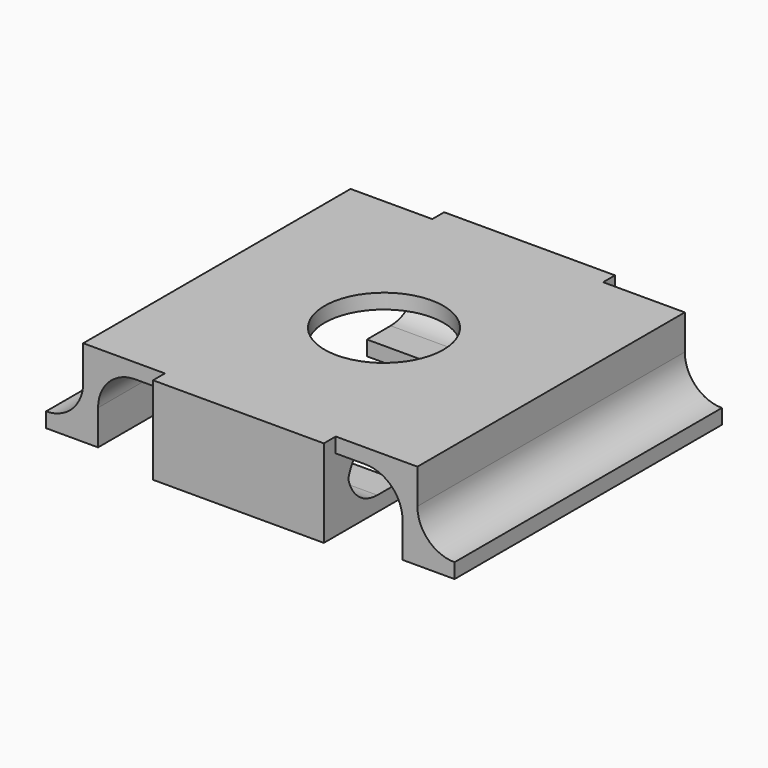
from build123d import *

# Parameters (mm, degrees)
F0_W         = 45
F0_H         = 45
F1_DEPTH     = 2
F2_R         = 8
F3_DEPTH     = 25
F4_W         = 23
F4_H         = 3.9995294809
F4_H_2       = 4
F5_DEPTH     = 9.8
F6_W         = 23
F6_H         = 9
F6_H_2       = 4
F7_DEPTH     = 2
F8_W         = 23
F8_H         = 13
F9_DEPTH     = 2
F10_W        = 2
F10_H        = 45
F11_DEPTH    = 7.7
F12_W        = 7
F12_H        = 45
F13_W        = 7
F13_H        = 45
F14_DEPTH    = 2
F15_T1_DEPTH = 23
F15_T3_DEPTH = 45


# Not quite as in the source:
# - a fillet or chamfer that OpenCascade refuses, or shapes differently, is made with other operations: its cross-section is extruded or revolved along the edge and cut away or added


with BuildPart() as f1:
    # F0 (on Top) → F1 (new body)
    with BuildSketch(Plane.XY):
        Rectangle(F0_W, F0_H)
    extrude(amount=F1_DEPTH)

    # F2 (on face) → F3 (cut)
    with BuildSketch(Plane.XY.offset(2)):
        Circle(F2_R)
    extrude(amount=-F3_DEPTH, mode=Mode.SUBTRACT)

    # F4 (on face) → F5 (join)
    with BuildSketch(Plane.XY.offset(2)):
        with Locations((0, 22.5)):
            Rectangle(F4_W, F4_H)
        with Locations((0, -22.5)):
            Rectangle(F4_W, F4_H_2)
    extrude(amount=-F5_DEPTH)

    # F6 (on face) → F7 (join)
    with BuildSketch(Plane(origin=(0, 0, -7.8), x_dir=(1, 0, 0), z_dir=(0, 0, -1))):
        with Locations((0, 16)):
            Rectangle(F6_W, F6_H)
        with Locations((0, 22.5)):
            Rectangle(F6_W, F6_H_2)
    extrude(amount=F7_DEPTH)

    # F8 (on face) → F9 (join)
    with BuildSketch(Plane(origin=(0, 0, -7.8), x_dir=(1, 0, 0), z_dir=(0, 0, -1))):
        with Locations((0, -17.9997647405)):
            Rectangle(F8_W, F8_H)
    extrude(amount=F9_DEPTH)

    # F10 (on face) → F11 (join)
    with BuildSketch(Plane(origin=(0, 0, 0), x_dir=(1, 0, 0), z_dir=(0, 0, -1))):
        with Locations((-21.5, 0)):
            Rectangle(F10_W, F10_H)
        with Locations((21.5, 0)):
            Rectangle(F10_W, F10_H)
    extrude(amount=F11_DEPTH)

    # F12 (on face) + F13 (on face) → F14 (join)
    with BuildSketch(Plane(origin=(0, 0, -7.7), x_dir=(1, 0, 0), z_dir=(0, 0, -1))):
        with Locations((-24, 0)):
            Rectangle(F12_W, F12_H)
    with BuildSketch(Plane(origin=(0, 0, -7.7), x_dir=(1, 0, 0), z_dir=(0, 0, -1))):
        with Locations((24, 0)):
            Rectangle(F13_W, F13_H)
    extrude(amount=F14_DEPTH)

    # F15: fillet of radius 5 on 8 edges, made by hand

    # F15_s2 → F15_t1 (join)
    with BuildSketch(Plane.YZ.offset(-11.5)):
        with BuildLine():
            ThreePointArc((-15.5, -7.8), (-19.0355339059, -6.3355339059), (-20.5, -2.8))
            Line((-20.5, -2.8), (-20.5, -7.8))
            Line((-20.5, -7.8), (-15.5, -7.8))
        make_face()
        with BuildLine():
            ThreePointArc((15.5002352595, -7.8), (19.0357691655, -6.3355339059), (20.5002352595, -2.8))
            Line((20.5002352595, -2.8), (20.5002352595, -7.8))
            Line((20.5002352595, -7.8), (15.5002352595, -7.8))
        make_face()
        with BuildLine():
            ThreePointArc((20.5002352595, -5), (19.0357691655, -1.4644660941), (15.5002352595, 0))
            Line((15.5002352595, 0), (20.5002352595, 0))
            Line((20.5002352595, 0), (20.5002352595, -5))
        make_face()
        with BuildLine():
            ThreePointArc((-20.5, -5), (-19.0355339059, -1.4644660941), (-15.5, 0))
            Line((-15.5, 0), (-20.5, 0))
            Line((-20.5, 0), (-20.5, -5))
        make_face()
    extrude(amount=F15_T1_DEPTH)

    # F15_s4 → F15_t3 (join)
    with BuildSketch(Plane.XZ.offset(-22.5)):
        with BuildLine():
            ThreePointArc((20.5, -5), (19.0355339059, -1.4644660941), (15.5, 0))
            Line((15.5, 0), (20.5, 0))
            Line((20.5, 0), (20.5, -5))
        make_face()
        with BuildLine():
            ThreePointArc((-20.5, -5), (-19.0355339059, -1.4644660941), (-15.5, 0))
            Line((-15.5, 0), (-20.5, 0))
            Line((-20.5, 0), (-20.5, -5))
        make_face()
        with BuildLine():
            ThreePointArc((-22.5, -2.7), (-23.9644660941, -6.2355339059), (-27.5, -7.7))
            Line((-27.5, -7.7), (-22.5, -7.7))
            Line((-22.5, -7.7), (-22.5, -2.7))
        make_face()
        with BuildLine():
            ThreePointArc((27.5, -7.7), (23.9644660941, -6.2355339059), (22.5, -2.7))
            Line((22.5, -2.7), (22.5, -7.7))
            Line((22.5, -7.7), (27.5, -7.7))
        make_face()
    extrude(amount=F15_T3_DEPTH)


solid = f1.part
